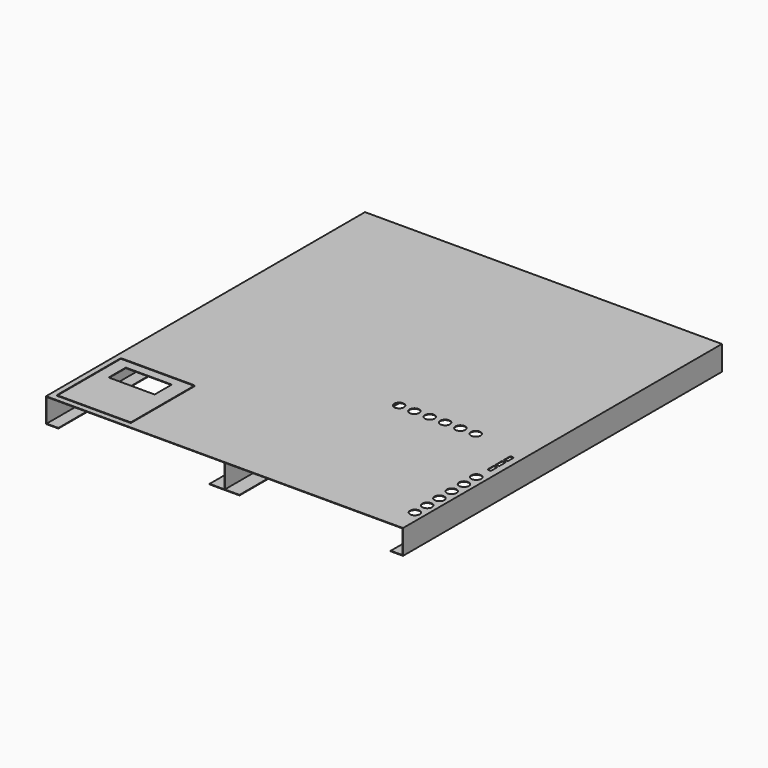
from build123d import *

# Parameters (mm, degrees)
F1_DEPTH = 325
F3_D     = 16
F3_DEPTH = 5
F3_TIP   = 4.8068849522
F2_W     = 6
F2_H     = 13
F2_W_2   = 75
F2_H_2   = 35
F4_DEPTH = 25
F6_DEPTH = 1
F8_DEPTH = 325


# Not quite as in the source:
# - a feature names something its author has since deleted; it is built from what else it names


with BuildPart() as f1:
    # F0 (on Front) → F1 (new body, symmetric)
    with BuildSketch(Plane.XZ):
        Polygon((-291, 20), (-291, -20), (-271, -20), (-271, -19.1), (-290.1, -19.1), (-290.1, 19.1), (290.1, 19.1), (290.1, -19.1), (271, -19.1), (271, -20), (291, -20), (291, 20), align=None)
    extrude(amount=F1_DEPTH, both=True)

    # F3
    with Locations(Plane.XY.offset(20)):
        with Locations((276, -282), (276, -257), (276, -232), (276, -207), (276, -182), (201, -64.213295877), (176, -64.213295877), (151, -64.213295877), (126, -64.213295877), (101, -64.213295877), (76, -64.213295877), (276, -157)):
            Hole(F3_D / 2, depth=F3_DEPTH)
            with Locations((0, 0, -(F3_DEPTH + F3_TIP / 2))):  # 118° drill point
                Cone(0, F3_D / 2, F3_TIP, mode=Mode.SUBTRACT)

    # F2 (on face) → F4 (cut)
    with BuildSketch(Plane.XY.offset(20)):
        with Locations((277, -125.5)):
            Rectangle(F2_W, F2_H)
        with Locations((-223.5, -217.5)):
            Rectangle(F2_W_2, F2_H_2)
        with Locations((277, -108.5)):
            Rectangle(F2_W, F2_H)
        with Locations((277, -91.5)):
            Rectangle(F2_W, F2_H)
    extrude(amount=-F4_DEPTH, mode=Mode.SUBTRACT)

    # F5 (on face) → F6 (join)
    with BuildSketch(Plane.XY.offset(20)):
        with BuildLine():
            Line((-161.5, -184.5), (-280.5, -184.5))
            ThreePointArc((-280.5, -184.5), (-281.2071067812, -184.7928932188), (-281.5, -185.5))
            Line((-281.5, -185.5), (-281.5, -314.5))
            ThreePointArc((-281.5, -314.5), (-281.2071067812, -315.2071067812), (-280.5, -315.5))
            Line((-280.5, -315.5), (-161.5, -315.5))
            ThreePointArc((-161.5, -315.5), (-160.7928932188, -315.2071067812), (-160.5, -314.5))
            Line((-160.5, -314.5), (-160.5, -185.5))
            ThreePointArc((-160.5, -185.5), (-160.7928932188, -184.7928932188), (-161.5, -184.5))
        make_face()
        with BuildLine():
            ThreePointArc((-281, -186), (-280.7071067812, -185.2928932188), (-280, -185))
            Line((-280, -185), (-162, -185))
            ThreePointArc((-162, -185), (-161.2928932188, -185.2928932188), (-161, -186))
            Line((-161, -186), (-161, -314))
            ThreePointArc((-161, -314), (-161.2928932188, -314.7071067812), (-162, -315))
            Line((-162, -315), (-280, -315))
            ThreePointArc((-280, -315), (-280.7071067812, -314.7071067812), (-281, -314))
            Line((-281, -314), (-281, -186))
        make_face(mode=Mode.SUBTRACT)
    extrude(amount=F6_DEPTH)

    # F7 (on Front) → F8 (join, symmetric)
    with BuildSketch(Plane.XZ):
        Polygon((-24.3627466261, -20), (24.3627466261, -20), (24.3627466261, -19.1), (0.4681956061, -19.1), (0.4681956061, 20), (-0.4318043939, 20), (-0.4318043939, -19.1), (-24.3627466261, -19.1), align=None)
    extrude(amount=F8_DEPTH, both=True)


solid = f1.part
